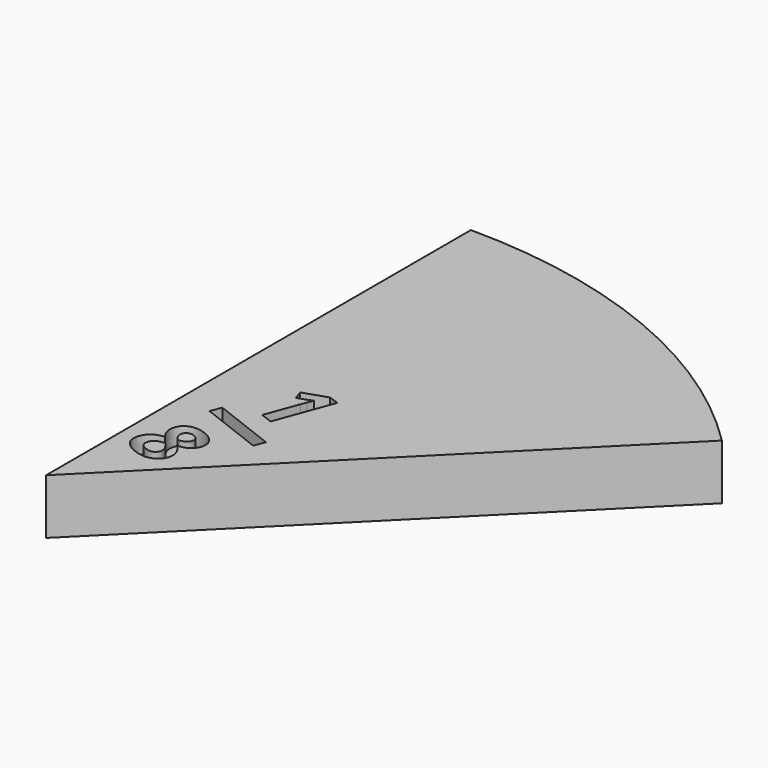
from build123d import *

# Parameters (mm, degrees)
F1_DEPTH     = 6.5
F2_R         = 12.5
F3_DEPTH     = 5
F4_TEXT_SIZE = 10.0164487022
F5_DEPTH     = 2
F7_DEPTH     = 2


# Not quite as in the source:
# - Text() gives the source's letters only with a copy of the font that has no kerning and outlines rounded to 1/6400 em; it was checked with that copy


with BuildPart() as f1:
    # F0 (on Top) → F1 (new body)
    with BuildSketch(Plane.XY):
        with BuildLine():
            Line((0, 0), (44.1941738242, 44.1941738242))
            ThreePointArc((44.1941738242, 44.1941738242), (23.9177145228, 57.742470782), (0, 62.5))
            Line((0, 62.5), (0, 0))
        make_face()
    extrude(amount=F1_DEPTH)

    # F2 (on face) → F3 (cut)
    with BuildSketch(Plane(origin=(0, 0, 0), x_dir=(1, 0, 0), z_dir=(0, 0, -1))):
        with Locations((17.9034210742, -42.5675660372)):
            Circle(F2_R)
    extrude(amount=-F3_DEPTH, mode=Mode.SUBTRACT)

    # F4 (on face) → F5 (cut)
    with BuildSketch(Plane.XY.offset(6.5)):
        with Locations(Location((5.5477601229, 22.6814797458), (0, 0, -20.1910068213))):
            Text('1', F4_TEXT_SIZE, font='Open Sans', font_style=FontStyle.BOLD, text_align=(TextAlign.LEFT, TextAlign.BOTTOM))
        with Locations(Location((0.845986935, 9.8962421762), (0, 0, -20.1910068213))):
            Text('8', F4_TEXT_SIZE, font='Open Sans', font_style=FontStyle.BOLD, text_align=(TextAlign.LEFT, TextAlign.BOTTOM))
    extrude(amount=-F5_DEPTH, mode=Mode.SUBTRACT)

    # F6 (on face) → F7 (cut)
    with BuildSketch(Plane.XY.offset(6.5)):
        Polygon((4.243563395, 20.6273812801), (3.7526518568, 19.3563911319), (11.1829232828, 16.4864979389), (11.673834821, 17.7574880871), align=None)
    extrude(amount=-F7_DEPTH, mode=Mode.SUBTRACT)


solid = f1.part
